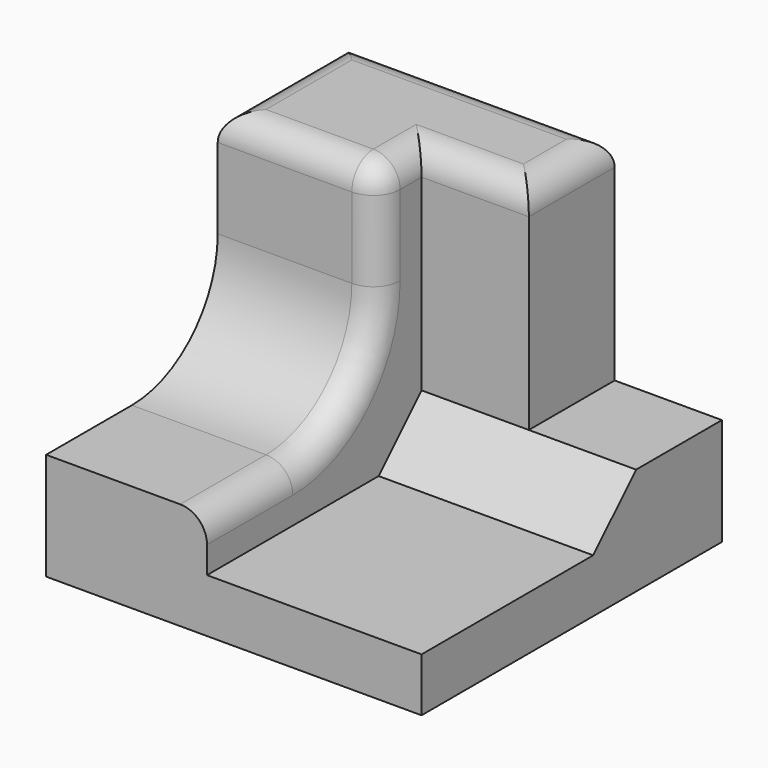
from build123d import *

# Parameters (mm, degrees)
F0_W          = 70
F0_H          = 70
F1_DEPTH      = 60
F3_DEPTH      = 70.001
F4_W          = 50
F4_H          = 50
F5_DEPTH      = 40
F6_SIZE       = 10
F7_W          = 20
F7_H          = 40
F8_DEPTH      = 20
F9_R          = 5
F10_T1_DEPTH  = 32.5
F10_T3_DEPTH  = 15
F10_S7_W      = 5
F10_S7_H      = 5
F10_T8_DEPTH  = 5
F10_T12_ANGLE = 90


# Not quite as in the source:
# - a fillet or chamfer that OpenCascade refuses, or shapes differently, is made with other operations: its cross-section is extruded or revolved along the edge and cut away or added


with BuildPart() as f1:
    # F0 (on Top) → F1 (new body)
    with BuildSketch(Plane.XY):
        with Locations((35, 35)):
            Rectangle(F0_W, F0_H)
    extrude(amount=F1_DEPTH)

    # F2 (on face) → F3 (cut, through all)
    with BuildSketch(Plane.YZ.offset(70)):
        with BuildLine():
            Line((40, 60), (0, 60))
            Line((0, 60), (0, 20))
            Line((0, 20), (20, 20))
            ThreePointArc((20, 20), (34.1421356237, 25.8578643763), (40, 40))
            Line((40, 40), (40, 60))
        make_face()
    extrude(amount=-F3_DEPTH, mode=Mode.SUBTRACT)

    # F4 (on face) → F5 (cut)
    with BuildSketch(Plane.YZ.offset(70)):
        with Locations((25, 35)):
            Rectangle(F4_W, F4_H)
    extrude(amount=-F5_DEPTH, mode=Mode.SUBTRACT)

    # F6
    f6_edges = [f1.edges().sort_by_distance(p)[0] for p in [
        (50, 50, 10),
    ]]
    chamfer(f6_edges, length=F6_SIZE)

    # F7 (on face) → F8 (cut)
    with BuildSketch(Plane.YZ.offset(70)):
        with Locations((60, 40)):
            Rectangle(F7_W, F7_H)
    extrude(amount=-F8_DEPTH, mode=Mode.SUBTRACT)

    # F9
    f9_edges = [f1.edges().sort_by_distance(p)[0] for p in [
        (40, 50, 60),
        (30, 45, 60),
        (15, 40, 60),
        (0, 55, 60),
        (25, 70, 60),
        (50, 60, 60),
    ]]
    fillet(f9_edges, radius=F9_R)

    # F10: fillet of radius 5 on 1 edges, made by hand

    # F10_s2 → F10_t1 (cut)
    with BuildSketch(Plane.XZ.offset(-20)):
        with BuildLine():
            ThreePointArc((25, 20), (28.5355339059, 18.5355339059), (30, 15))
            Line((30, 15), (30, 20))
            Line((30, 20), (25, 20))
        make_face()
    extrude(amount=F10_T1_DEPTH, mode=Mode.SUBTRACT)

    # F10_s4 → F10_t3 (cut)
    with BuildSketch(Plane.XY.offset(40)):
        with BuildLine():
            ThreePointArc((25, 40), (28.5355339059, 41.4644660941), (30, 45))
            Line((30, 45), (30, 40))
            Line((30, 40), (25, 40))
        make_face()
    extrude(amount=F10_T3_DEPTH, mode=Mode.SUBTRACT)


with BuildPart() as f10_tool6:
    # F10_s7 → F10_t8 (new body)
    with BuildSketch(Plane.XZ.offset(-45)):
        with Locations((27.5, 57.5)):
            Rectangle(F10_S7_W, F10_S7_H)
    extrude(amount=F10_T8_DEPTH)

    # F10_s9 → F10_t10 (revolve, cut)
    with BuildSketch(Plane(origin=(25, 45, 55), x_dir=(-0.7071067812, 0, -0.7071067812), z_dir=(-0.7071067812, 0, 0.7071067812))):
        with BuildLine():
            ThreePointArc((0, -5), (5, 0), (0, 5))
            Line((0, 5), (0, -5))
        make_face()
    revolve(axis=Axis((25, 45, 55), (0, -1, 0)), mode=Mode.SUBTRACT)


with BuildPart() as f1_1:
    add(f1.part)

    # F10_t5: cut F10_tool6
    add(f10_tool6.part, mode=Mode.SUBTRACT)

    # F10_s11 → F10_t12 (revolve, cut)
    with BuildSketch(Plane.XZ.offset(-20)):
        with BuildLine():
            ThreePointArc((25, 20), (28.5355339059, 18.5355339059), (30, 15))
            Line((30, 15), (30, 20))
            Line((30, 20), (25, 20))
        make_face()
    revolve(axis=Axis((30, 20, 40), (1, 0, 0)), revolution_arc=F10_T12_ANGLE, mode=Mode.SUBTRACT)


solid = f1_1.part
